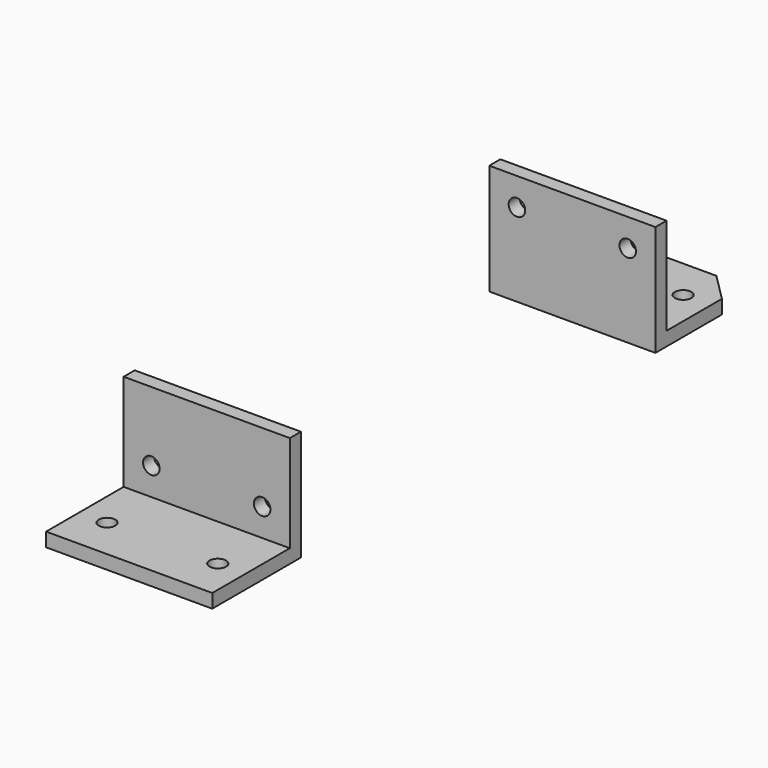
from build123d import *

# Parameters (mm, degrees)
F0_W      = 38.1
F0_H      = 3.175
F1_DEPTH  = 25.4
F2_W      = 3.175
F2_H      = 22.225
F3_DEPTH  = 38.1
F5_D      = 3.7973
F5_DEPTH  = 12.7
F5_TIP    = 1.1408240143
F7_D      = 3.7973
F7_DEPTH  = 12.7
F7_TIP    = 1.1408240143
F10_R     = 3.3782
F10_R_2   = 1.89865
F11_DEPTH = 3.175
F14_D     = 3.7973
F14_DEPTH = 12.7
F14_TIP   = 1.1408240143
F15_R     = 1.89865
F16_DEPTH = 3.175
F18_DEPTH = 25.4


with BuildPart() as f1:
    # F0 (on Front) → F1 (new body)
    with BuildSketch(Plane.XZ):
        with Locations((19.05, -1.5875)):
            Rectangle(F0_W, F0_H)
    extrude(amount=F1_DEPTH)

    # F2 (on face) → F3 (join)
    with BuildSketch(Plane.YZ.offset(38.1)):
        with Locations((-23.8125, 11.1125)):
            Rectangle(F2_W, F2_H)
    extrude(amount=-F3_DEPTH)

    # F5
    with Locations(Plane.XZ.offset(25.4)):
        with Locations((6.35, 15.875), (31.75, 15.875)):
            Hole(F5_D / 2, depth=F5_DEPTH)
            with Locations((0, 0, -(F5_DEPTH + F5_TIP / 2))):  # 118° drill point
                Cone(0, F5_D / 2, F5_TIP, mode=Mode.SUBTRACT)

    # F7
    with Locations(Plane(origin=(0, 0, -3.175), x_dir=(1, 0, 0), z_dir=(0, 0, -1))):
        with Locations((6.35, 9.525), (31.75, 9.525)):
            Hole(F7_D / 2, depth=F7_DEPTH)
            with Locations((0, 0, -(F7_DEPTH + F7_TIP / 2))):  # 118° drill point
                Cone(0, F7_D / 2, F7_TIP, mode=Mode.SUBTRACT)


with BuildPart() as f9_1:
    # F9: instance of F1
    add(f1.part.mirror(Plane(origin=(19.05, -76.2, 9.3728155466), x_dir=(1, 0, 0), z_dir=(0, -1, 0))))


with BuildPart() as f11:
    # F10 (on face) → F11 (new body)
    with BuildSketch(Plane.XZ.offset(130.175)):
        with Locations((6.35, 15.875)):
            Circle(F10_R)
        with Locations((6.35, 15.875)):
            Circle(F10_R_2, mode=Mode.SUBTRACT)
    extrude(amount=-F11_DEPTH)

    # F12: union F9_1
    add(f9_1.part)

    # F14
    with Locations(Plane.XZ.offset(130.175)):
        with Locations((31.75, 6.35), (6.35, 6.35)):
            Hole(F14_D / 2, depth=F14_DEPTH)
            with Locations((0, 0, -(F14_DEPTH + F14_TIP / 2))):  # 118° drill point
                Cone(0, F14_D / 2, F14_TIP, mode=Mode.SUBTRACT)

    # F15 (on face) → F16 (join)
    with BuildSketch(Plane.XZ.offset(130.175)):
        with Locations((6.35, 15.875)):
            Circle(F15_R)
        with Locations((31.75, 15.875)):
            Circle(F15_R)
    extrude(amount=-F16_DEPTH)


with BuildPart() as f1_1:
    add(f1.part)

    # F17 (on face) → F18 (cut)
    with BuildSketch(Plane.XY):
        Polygon((6.35, 0), (0, 0), (0, -6.35), align=None)
        Polygon((38.1, 0), (31.75, 0), (38.1, -6.35), align=None)
    extrude(amount=-F18_DEPTH, mode=Mode.SUBTRACT)


solid = Compound([f11.part, f1_1.part])
